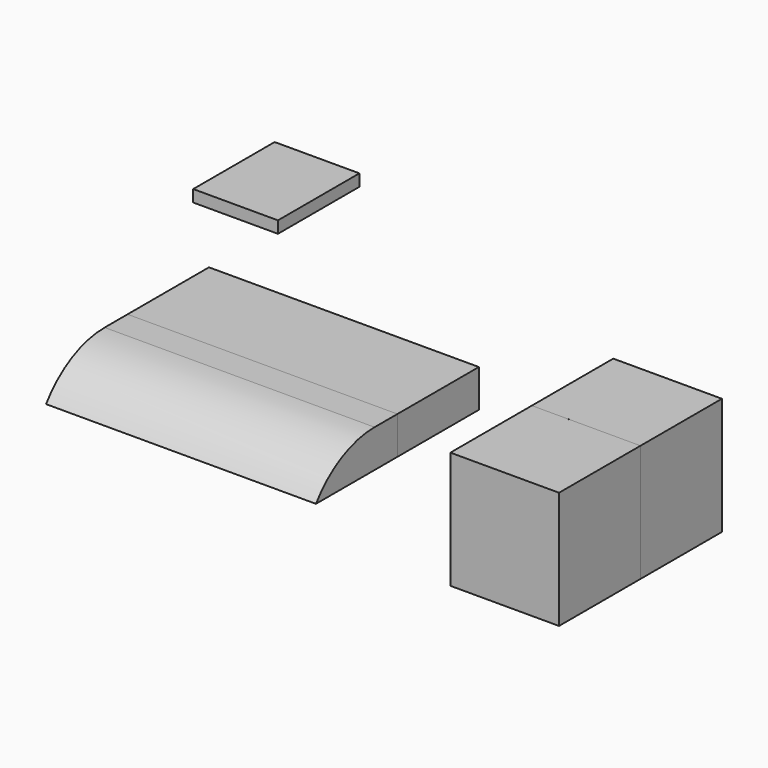
from build123d import *

# Parameters (mm, degrees)
F0_W        = 67.3399567604
F0_H        = 9.4070211053
F1_DEPTH    = 25.4
F0_W_2      = 21.1403407156
F0_H_2      = 2.9615163803
F0_W_3      = 27.1071493626
F0_H_3      = 29.2595624924
F2_DEPTH    = 25.4
F3_T1_DEPTH = 158.6723585187


# Not quite as in the source:
# - a fillet or chamfer that OpenCascade refuses, or shapes differently, is made with other operations: its cross-section is extruded or revolved along the edge and cut away or added


with BuildPart() as f1:
    # F0 (on Front) → F1 (new body)
    with BuildSketch(Plane.XZ):
        with Locations((-33.6699783802, -52.3458756506)):
            Rectangle(F0_W, F0_H)
    extrude(amount=F1_DEPTH)


with BuildPart() as f1b:
    # F0 (on Front) → F1, piece 2 (new body)
    with BuildSketch(Plane.XZ):
        with Locations((-40.380159393, -16.2786431611)):
            Rectangle(F0_W_2, F0_H_2)
    extrude(amount=F1_DEPTH)


with BuildPart() as f1c:
    # F0 (on Front) → F1, piece 3 (new body)
    with BuildSketch(Plane.XZ):
        with Locations((47.0881126821, -49.5216473937)):
            Rectangle(F0_W_3, F0_H_3)
    extrude(amount=F1_DEPTH)


with BuildPart() as f2:
    # F2 (new): a face of the model
    f2_faces = [f1c.part.faces().sort_by_distance(p)[0] for p in [
        (47.0881126821, -25.4, -49.5216473937),
    ]]
    extrude(f2_faces, amount=F2_DEPTH)


with BuildPart() as f2b:
    # F2#2 (new): a face of the model
    f2_2_faces = [f1.part.faces().sort_by_distance(p)[0] for p in [
        (-33.6699783802, -25.4, -52.3458756506),
    ]]
    extrude(f2_2_faces, amount=F2_DEPTH)

    # F3: fillet of radius 22.4383652268 on 1 edges, made by hand

    # F3_s2 → F3_t1 (cut)
    with BuildSketch(Plane.YZ.offset(-113.0061576395)):
        with BuildLine():
            ThreePointArc((-32.5335196483, -47.642365098), (-42.8067415202, -50.1322680677), (-50.8, -57.0493862033))
            Line((-50.8, -57.0493862033), (-50.8, -47.642365098))
            Line((-50.8, -47.642365098), (-32.5335196483, -47.642365098))
        make_face()
    extrude(amount=F3_T1_DEPTH, mode=Mode.SUBTRACT)


solid = Compound([f1.part, f1b.part, f1c.part, f2.part, f2b.part])
